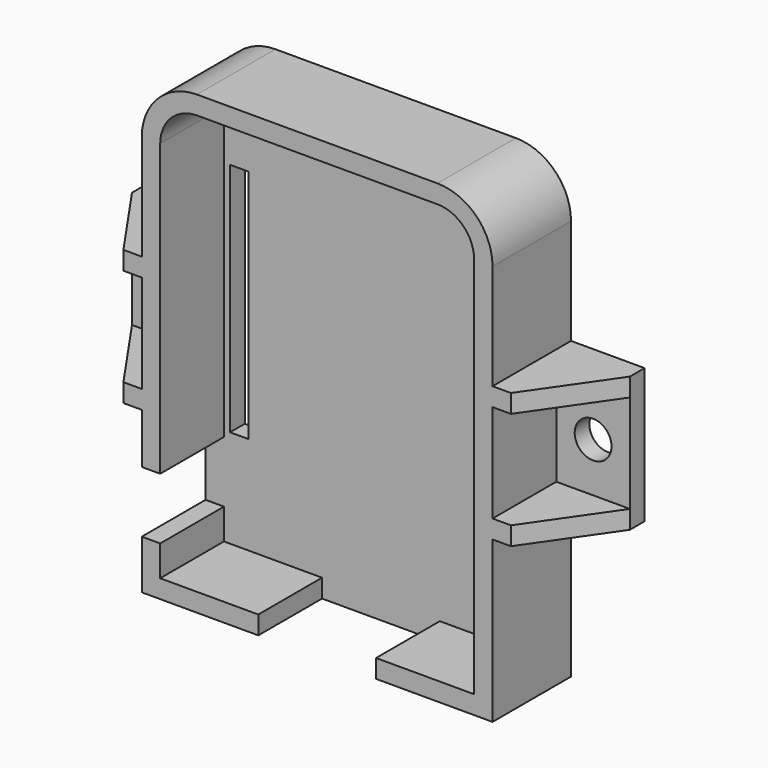
from build123d import *

# Parameters (mm, degrees)
F0_W      = 6
F0_H      = 1.5
F1_DEPTH  = 8
F0_H_2    = 8
F0_R      = 1.5
F2_DEPTH  = 1.5
F4_DEPTH  = 25
F6_DEPTH  = 25
F7_W      = 9.6
F7_H      = 6.5
F8_DEPTH  = 1.5
F9_W      = 6.5
F9_H      = 5
F10_DEPTH = 1.5
F11_W     = 1.5
F11_H     = 19.2
F12_DEPTH = 1.5


# Not quite as in the source:
# - a feature names something its author has since deleted; it is built from what else it names


with BuildPart() as f1:
    # F0 (on Front) → F1 (new body)
    with BuildSketch(Plane.XZ):
        with Locations((4.5, 12.35)):
            Rectangle(F0_W, F0_H)
        with Locations((4.5, 21.85)):
            Rectangle(F0_W, F0_H)
        with Locations((-30.1, 12.35)):
            Rectangle(F0_W, F0_H)
        with Locations((-30.1, 21.85)):
            Rectangle(F0_W, F0_H)
        with BuildLine():
            Line((-27.1, 11.6), (-27.1, -1.5))
            Line((-27.1, -1.5), (1.5, -1.5))
            Line((1.5, -1.5), (1.5, 11.6))
            Line((1.5, 11.6), (1.5, 13.1))
            Line((1.5, 13.1), (1.5, 21.1))
            Line((1.5, 21.1), (1.5, 22.6))
            Line((1.5, 22.6), (1.5, 31.2))
            ThreePointArc((1.5, 31.2), (0.1819805153, 34.3819805153), (-3, 35.7))
            Line((-3, 35.7), (-22.6, 35.7))
            ThreePointArc((-22.6, 35.7), (-25.7819805153, 34.3819805153), (-27.1, 31.2))
            Line((-27.1, 31.2), (-27.1, 22.6))
            Line((-27.1, 22.6), (-27.1, 21.1))
            Line((-27.1, 21.1), (-27.1, 13.1))
            Line((-27.1, 13.1), (-27.1, 11.6))
        make_face()
        with BuildLine():
            ThreePointArc((-25.6, 31.2), (-24.7213203436, 33.3213203436), (-22.6, 34.2))
            Line((-22.6, 34.2), (-3, 34.2))
            ThreePointArc((-3, 34.2), (-0.8786796564, 33.3213203436), (0, 31.2))
            Line((0, 31.2), (0, 0))
            Line((0, 0), (-25.6, 0))
            Line((-25.6, 0), (-25.6, 31.2))
        make_face(mode=Mode.SUBTRACT)
    extrude(amount=F1_DEPTH)

    # F0 (on Front) → F2 (join)
    with BuildSketch(Plane.XZ):
        with Locations((4.5, 17.1)):
            Rectangle(F0_W, F0_H_2)
        with Locations((4.5, 17.1)):
            Circle(F0_R, mode=Mode.SUBTRACT)
        with Locations((-30.1, 17.1)):
            Rectangle(F0_W, F0_H_2)
        with Locations((-30.1, 17.1)):
            Circle(F0_R, mode=Mode.SUBTRACT)
        with BuildLine():
            Line((-3, 34.2), (-22.6, 34.2))
            ThreePointArc((-22.6, 34.2), (-24.7213203436, 33.3213203436), (-25.6, 31.2))
            Line((-25.6, 31.2), (-25.6, 0))
            Line((-25.6, 0), (0, 0))
            Line((0, 0), (0, 31.2))
            ThreePointArc((0, 31.2), (-0.8786796564, 33.3213203436), (-3, 34.2))
        make_face()
    extrude(amount=F2_DEPTH)

    # F3 (on face) → F4 (cut)
    with BuildSketch(Plane(origin=(0, 0, 11.6), x_dir=(1, 0, 0), z_dir=(0, 0, -1))):
        Polygon((7.5, 8), (3, 8), (7.5, 1.5), align=None)
    extrude(amount=-F4_DEPTH, mode=Mode.SUBTRACT)

    # F5 (on face) → F6 (cut)
    with BuildSketch(Plane(origin=(0, 0, 11.6), x_dir=(1, 0, 0), z_dir=(0, 0, -1))):
        Polygon((-33.1, 1.5), (-28.6, 8), (-33.1, 8), align=None)
    extrude(amount=-F6_DEPTH, mode=Mode.SUBTRACT)

    # F7 (on face) → F8 (cut, through all)
    with BuildSketch(Plane(origin=(0, 0, -1.5), x_dir=(1, 0, 0), z_dir=(0, 0, -1))):
        with Locations((-12.8, 4.75)):
            Rectangle(F7_W, F7_H)
    extrude(amount=-F8_DEPTH, mode=Mode.SUBTRACT)

    # F9 (on face) → F10 (cut, through all)
    with BuildSketch(Plane(origin=(-27.1, 0, 0), x_dir=(0, -1, 0), z_dir=(-1, 0, 0))):
        with Locations((4.75, 5)):
            Rectangle(F9_W, F9_H)
    extrude(amount=-F10_DEPTH, mode=Mode.SUBTRACT)

    # F11 (on face) → F12 (cut, through all)
    with BuildSketch(Plane.XZ.offset(1.5)):
        with Locations((-24.35, 17.6)):
            Rectangle(F11_W, F11_H)
        with Locations((-1.25, 17.6)):
            Rectangle(F11_W, F11_H)
    extrude(amount=-F12_DEPTH, mode=Mode.SUBTRACT)


solid = f1.part
